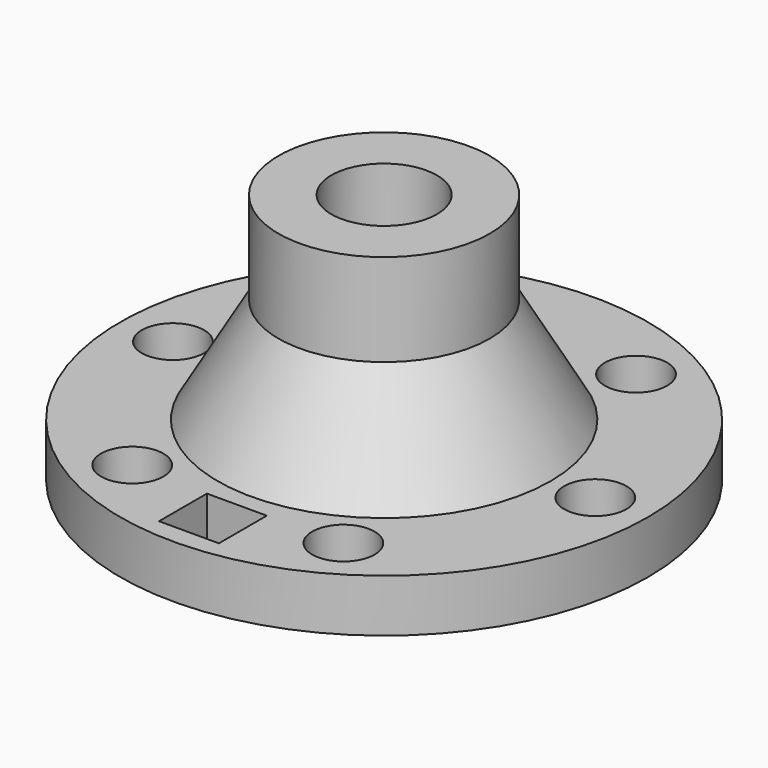
from build123d import *

# Parameters (mm, degrees)
F2_R            = 7.5
F3_DEPTH        = 12.701
F3_COPIES_COUNT = 6
F4_W            = 14.403924346
F4_H            = 14.403924346
F5_DEPTH        = 12.701


# Not quite as in the source:
# - a pattern or mirror of a feature is missing from the dataset's text; its kind, count and spacing are read off the source's solid


with BuildPart() as f1:
    # F0 (on Front) → F1 (revolve)
    with BuildSketch(Plane.XZ):
        Polygon((25.4, 60.325), (12.7, 60.325), (12.7, 34.6970452561), (32.7323484187, 0), (63.5, 0), (63.5, 12.7), (40.0646968374, 12.7), (25.4, 38.1), align=None)
    revolve(axis=Axis((0, 0, 18.9653343184), (0, 0, 1)))

    # F2 (on face) → F3 (cut, through all)
    with BuildSketch(Plane.XY.offset(12.7)):
        with Locations((-50.8, 0)):
            Circle(F2_R)
    f3 = extrude(amount=-F3_DEPTH, mode=Mode.SUBTRACT)

    # F3_copies: F3 ×6 about axis
    f3_copies_axis = Axis((0, 0, 0), (0, 0, 1))
    for i in range(1, F3_COPIES_COUNT):
        add(f3.rotate(f3_copies_axis, i * 360 / F3_COPIES_COUNT), mode=Mode.SUBTRACT)

    # F4 (on face) → F5 (cut, through all)
    with BuildSketch(Plane.XY.offset(12.7)):
        with Locations((0, -51.4825247228)):
            Rectangle(F4_W, F4_H)
    extrude(amount=-F5_DEPTH, mode=Mode.SUBTRACT)


solid = f1.part
